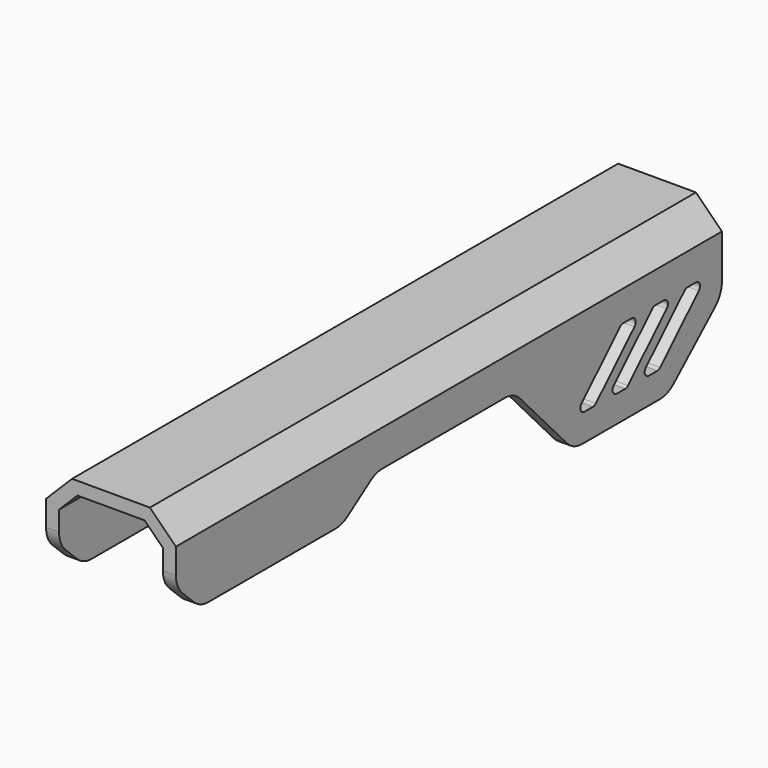
from build123d import *

# Parameters (mm, degrees)
F1_DEPTH     = 12.5
F2_SIZE      = 5
F3_T         = -2.5
F4_T1_DEPTH  = 2.5
F4_T3_DEPTH  = 2.5
F4_T5_DEPTH  = 2.5
F4_T7_DEPTH  = 2.5
F4_T9_DEPTH  = 13.1824295502
F4_T11_DEPTH = 13.1824295502
F4_T13_DEPTH = 12.5312469121
F4_T15_DEPTH = 12.5312469121
F4_T17_DEPTH = 10.2199869631
F4_T19_DEPTH = 10.2199869631
F4_T21_DEPTH = 13.4131081399
F4_T23_DEPTH = 13.4131081399
F4_T25_DEPTH = 12.0794727567
F4_T27_DEPTH = 12.0794727567
F4_T29_DEPTH = 13.6486136239
F4_T31_DEPTH = 13.6486136239
F6_DEPTH     = 12.5
F7_R         = 1


# Not quite as in the source:
# - a fillet or chamfer that OpenCascade refuses, or shapes differently, is made with other operations: its cross-section is extruded or revolved along the edge and cut away or added


with BuildPart() as f1:
    # F0 (on Right) → F1 (new body, symmetric)
    with BuildSketch(Plane.YZ):
        Polygon((64.5619183779, 36.750972271), (-66.8933242559, 36.750972271), (-66.8933242559, 24.738561362), (-61.0711984336, 19.1697143018), (-26.9197300076, 19.1697143018), (-18.7147669494, 24.7712358832), (14.4842416048, 24.7712358832), (28.7493690848, 9.385228157), (51.5191629529, 9.385228157), (64.5619183779, 21.1007967591), align=None)
    extrude(amount=F1_DEPTH, both=True)

    # F2
    f2_edges = [f1.edges().sort_by_distance(p)[0] for p in [
        (12.5, -1.165703, 36.750972),
        (-12.5, -1.165703, 36.750972),
    ]]
    chamfer(f2_edges, length=F2_SIZE)

    # F3
    f3_openings = [f1.faces().sort_by_distance(p)[0] for p in [
        (0, -66.893324, 30.350708),
        (0, -63.982261, 21.954138),
        (0, -43.995464, 19.169714),
        (0, -22.817248, 21.970475),
        (0, -2.115263, 24.771236),
        (0, 21.616805, 17.078232),
        (0, 40.134266, 9.385228),
        (0, 58.040541, 15.243012),
        (0, 64.561918, 28.50552),
    ]]
    offset(amount=F3_T, openings=f3_openings)

    # F4: fillet of radius 5 on 22 edges, made by hand

    # F4_s2 → F4_t1 (join)
    with BuildSketch(Plane.YZ.offset(-12.5)):
        with BuildLine():
            ThreePointArc((-19.9899366893, 23.9006785429), (-18.6460299918, 24.5486417325), (-17.1707695568, 24.7712358832))
            Line((-17.1707695568, 24.7712358832), (-18.7147669494, 24.7712358832))
            Line((-18.7147669494, 24.7712358832), (-19.9899366893, 23.9006785429))
        make_face()
    extrude(amount=F4_T1_DEPTH)

    # F4_s4 → F4_t3 (join)
    with BuildSketch(Plane.YZ.offset(10)):
        with BuildLine():
            ThreePointArc((-19.9899366893, 23.9006785429), (-18.6460299918, 24.5486417325), (-17.1707695568, 24.7712358832))
            Line((-17.1707695568, 24.7712358832), (-18.7147669494, 24.7712358832))
            Line((-18.7147669494, 24.7712358832), (-19.9899366893, 23.9006785429))
        make_face()
    extrude(amount=F4_T3_DEPTH)

    # F4_s6 → F4_t5 (join)
    with BuildSketch(Plane.YZ.offset(-12.5)):
        with BuildLine():
            ThreePointArc((12.3016199768, 24.7712358832), (14.3019608026, 24.3536628145), (15.9681862456, 23.1706905155))
            Line((15.9681862456, 23.1706905155), (14.4842416048, 24.7712358832))
            Line((14.4842416048, 24.7712358832), (12.3016199768, 24.7712358832))
        make_face()
    extrude(amount=F4_T5_DEPTH)

    # F4_s8 → F4_t7 (join)
    with BuildSketch(Plane.YZ.offset(10)):
        with BuildLine():
            ThreePointArc((12.3016199768, 24.7712358832), (14.3019608026, 24.3536628145), (15.9681862456, 23.1706905155))
            Line((15.9681862456, 23.1706905155), (14.4842416048, 24.7712358832))
            Line((14.4842416048, 24.7712358832), (12.3016199768, 24.7712358832))
        make_face()
    extrude(amount=F4_T7_DEPTH)

    # F4_s10 → F4_t9 (cut)
    with BuildSketch(Plane.YZ.offset(-17.8412147751)):
        with BuildLine():
            ThreePointArc((-66.8933242559, 26.8750472721), (-66.4911680254, 24.9104015861), (-65.3493911873, 23.2617937014))
            Line((-65.3493911873, 23.2617937014), (-66.8933242559, 24.738561362))
            Line((-66.8933242559, 24.738561362), (-66.8933242559, 26.8750472721))
        make_face()
    extrude(amount=F4_T9_DEPTH, mode=Mode.SUBTRACT)

    # F4_s12 → F4_t11 (cut)
    with BuildSketch(Plane.YZ.offset(4.6587852249)):
        with BuildLine():
            ThreePointArc((-66.8933242559, 26.8750472721), (-66.4911680254, 24.9104015861), (-65.3493911873, 23.2617937014))
            Line((-65.3493911873, 23.2617937014), (-66.8933242559, 24.738561362))
            Line((-66.8933242559, 24.738561362), (-66.8933242559, 26.8750472721))
        make_face()
    extrude(amount=F4_T11_DEPTH, mode=Mode.SUBTRACT)

    # F4_s14 → F4_t13 (cut)
    with BuildSketch(Plane.YZ.offset(-17.5156234561)):
        with BuildLine():
            ThreePointArc((-59.0649490512, 19.1697143018), (-60.9269012722, 19.5293335064), (-62.5210159826, 20.5564607312))
            Line((-62.5210159826, 20.5564607312), (-61.0711984336, 19.1697143018))
            Line((-61.0711984336, 19.1697143018), (-59.0649490512, 19.1697143018))
        make_face()
    extrude(amount=F4_T13_DEPTH, mode=Mode.SUBTRACT)

    # F4_s16 → F4_t15 (cut)
    with BuildSketch(Plane.YZ.offset(4.9843765439)):
        with BuildLine():
            ThreePointArc((-59.0649490512, 19.1697143018), (-60.9269012722, 19.5293335064), (-62.5210159826, 20.5564607312))
            Line((-62.5210159826, 20.5564607312), (-61.0711984336, 19.1697143018))
            Line((-61.0711984336, 19.1697143018), (-59.0649490512, 19.1697143018))
        make_face()
    extrude(amount=F4_T15_DEPTH, mode=Mode.SUBTRACT)

    # F4_s18 → F4_t17 (cut)
    with BuildSketch(Plane.YZ.offset(-16.3599934815)):
        with BuildLine():
            ThreePointArc((-25.6445602678, 20.0402716422), (-26.9884669653, 19.3923084525), (-28.4637274003, 19.1697143018))
            Line((-28.4637274003, 19.1697143018), (-26.9197300076, 19.1697143018))
            Line((-26.9197300076, 19.1697143018), (-25.6445602678, 20.0402716422))
        make_face()
    extrude(amount=F4_T17_DEPTH, mode=Mode.SUBTRACT)

    # F4_s20 → F4_t19 (cut)
    with BuildSketch(Plane.YZ.offset(6.1400065185)):
        with BuildLine():
            ThreePointArc((-25.6445602678, 20.0402716422), (-26.9884669653, 19.3923084525), (-28.4637274003, 19.1697143018))
            Line((-28.4637274003, 19.1697143018), (-26.9197300076, 19.1697143018))
            Line((-26.9197300076, 19.1697143018), (-25.6445602678, 20.0402716422))
        make_face()
    extrude(amount=F4_T19_DEPTH, mode=Mode.SUBTRACT)

    # F4_s22 → F4_t21 (cut)
    with BuildSketch(Plane.YZ.offset(-17.9565540699)):
        with BuildLine():
            ThreePointArc((30.9319907128, 9.385228157), (28.931649887, 9.8028012257), (27.2654244441, 10.9857735247))
            Line((27.2654244441, 10.9857735247), (28.7493690848, 9.385228157))
            Line((28.7493690848, 9.385228157), (30.9319907128, 9.385228157))
        make_face()
    extrude(amount=F4_T21_DEPTH, mode=Mode.SUBTRACT)

    # F4_s24 → F4_t23 (cut)
    with BuildSketch(Plane.YZ.offset(4.5434459301)):
        with BuildLine():
            ThreePointArc((30.9319907128, 9.385228157), (28.931649887, 9.8028012257), (27.2654244441, 10.9857735247))
            Line((27.2654244441, 10.9857735247), (28.7493690848, 9.385228157))
            Line((28.7493690848, 9.385228157), (30.9319907128, 9.385228157))
        make_face()
    extrude(amount=F4_T23_DEPTH, mode=Mode.SUBTRACT)

    # F4_s26 → F4_t25 (cut)
    with BuildSketch(Plane.YZ.offset(-17.2897363783)):
        with BuildLine():
            ThreePointArc((52.9444804464, 10.6655101473), (51.3923198194, 9.7162566403), (49.6032684016, 9.385228157))
            Line((49.6032684016, 9.385228157), (51.5191629529, 9.385228157))
            Line((51.5191629529, 9.385228157), (52.9444804464, 10.6655101473))
        make_face()
    extrude(amount=F4_T25_DEPTH, mode=Mode.SUBTRACT)

    # F4_s28 → F4_t27 (cut)
    with BuildSketch(Plane.YZ.offset(5.2102636217)):
        with BuildLine():
            ThreePointArc((52.9444804464, 10.6655101473), (51.3923198194, 9.7162566403), (49.6032684016, 9.385228157))
            Line((49.6032684016, 9.385228157), (51.5191629529, 9.385228157))
            Line((51.5191629529, 9.385228157), (52.9444804464, 10.6655101473))
        make_face()
    extrude(amount=F4_T27_DEPTH, mode=Mode.SUBTRACT)

    # F4_s30 → F4_t29 (cut)
    with BuildSketch(Plane.YZ.offset(4.425693188)):
        with BuildLine():
            ThreePointArc((64.5619183779, 23.3305194839), (64.128430188, 21.2941084527), (62.9031304227, 19.6108014742))
            Line((62.9031304227, 19.6108014742), (64.5619183779, 21.1007967591))
            Line((64.5619183779, 21.1007967591), (64.5619183779, 23.3305194839))
        make_face()
    extrude(amount=F4_T29_DEPTH, mode=Mode.SUBTRACT)

    # F4_s32 → F4_t31 (cut)
    with BuildSketch(Plane.YZ.offset(-18.074306812)):
        with BuildLine():
            ThreePointArc((64.5619183779, 23.3305194839), (64.128430188, 21.2941084527), (62.9031304227, 19.6108014742))
            Line((62.9031304227, 19.6108014742), (64.5619183779, 21.1007967591))
            Line((64.5619183779, 21.1007967591), (64.5619183779, 23.3305194839))
        make_face()
    extrude(amount=F4_T31_DEPTH, mode=Mode.SUBTRACT)

    # F5 (on Right) → F6 (cut, symmetric)
    with BuildSketch(Plane.YZ):
        Polygon((49.3934080005, 14.4370365888), (60.7276931405, 25.6640575826), (55.865034461, 25.6640575826), (44.530749321, 14.4370365888), align=None)
        Polygon((48.1250985598, 25.7630067087), (36.7908134197, 14.5359857149), (41.6534720992, 14.5359857149), (52.9877572393, 25.7630067087), align=None)
        Polygon((40.3851626585, 25.8619558348), (29.0508775185, 14.6349348409), (33.913536198, 14.6349348409), (45.247821338, 25.8619558348), align=None)
    extrude(amount=F6_DEPTH, both=True, mode=Mode.SUBTRACT)

    # F7
    f7_edges = [f1.edges().sort_by_distance(p)[0] for p in [
        (-11.25, 60.727693, 25.664058),
        (-11.25, 55.865034, 25.664058),
        (-11.25, 44.530749, 14.437037),
        (-11.25, 36.790813, 14.535986),
        (-11.25, 29.050878, 14.634935),
        (-11.25, 49.393408, 14.437037),
        (-11.25, 41.653472, 14.535986),
        (-11.25, 33.913536, 14.634935),
        (-11.25, 52.987757, 25.763007),
        (-11.25, 45.247821, 25.861956),
        (-11.25, 40.385163, 25.861956),
        (-11.25, 48.125099, 25.763007),
        (11.25, 60.727693, 25.664058),
        (11.25, 52.987757, 25.763007),
        (11.25, 45.247821, 25.861956),
        (11.25, 49.393408, 14.437037),
        (11.25, 41.653472, 14.535986),
        (11.25, 33.913536, 14.634935),
        (11.25, 40.385163, 25.861956),
        (11.25, 48.125099, 25.763007),
        (11.25, 55.865034, 25.664058),
        (11.25, 29.050878, 14.634935),
        (11.25, 36.790813, 14.535986),
        (11.25, 44.530749, 14.437037),
    ]]
    fillet(f7_edges, radius=F7_R)


solid = f1.part
